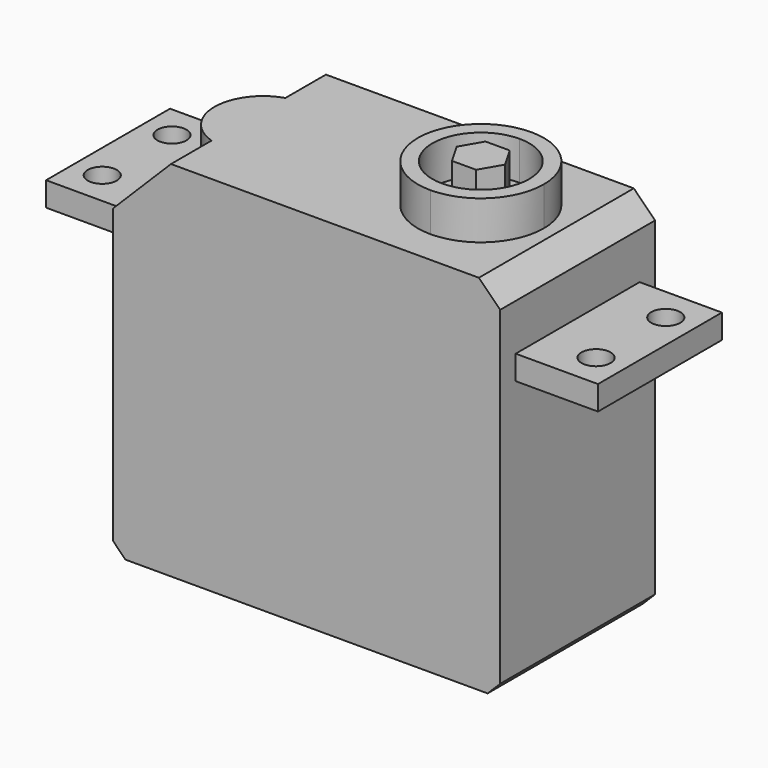
from build123d import *

# Parameters (mm, degrees)
F1_DEPTH    = 14
F2_DEPTH    = 13.5
F0_R        = 9.5
F3_DEPTH    = 9.5
F4_DEPTH    = 9.5
F5_DEPTH    = 28
F0_R_2      = 1.5
F6_DEPTH    = 2.5
F7_SIZE     = 2.2
F8_T1_DEPTH = 50.8601958556
F9_DEPTH    = 9.5
F10_SIZE    = 1.3


# Not quite as in the source:
# - a fillet or chamfer that OpenCascade refuses, or shapes differently, is made with other operations: its cross-section is extruded or revolved along the edge and cut away or added


with BuildPart() as f1:
    # F0 (on Top) → F1 (new body)
    with BuildSketch(Plane.XY):
        Polygon((10, 2.1650635095), (8.75, 2.1650635095), (7.5, 0), (8.75, -2.1650635095), (10, -2.1650635095), (10, 0), align=None)
        Polygon((11.25, 2.1650635095), (10, 2.1650635095), (10, 0), (10, -2.1650635095), (11.25, -2.1650635095), (12.5, 0), align=None)
    extrude(amount=F1_DEPTH)



with BuildPart() as f2:
    # F0 (on Top) → F2 (new body)
    with BuildSketch(Plane.XY):
        with BuildLine():
            ThreePointArc((10, -5), (5, 0), (10, 5))
            Line((10, 5), (10, 6.5))
            ThreePointArc((10, 6.5), (3.5, 0), (10, -6.5))
            Line((10, -6.5), (10, -5))
        make_face()
        with BuildLine():
            Line((10, 6.5), (10, 5))
            ThreePointArc((10, 5), (13.5355339059, 3.5355339059), (15, 0))
            ThreePointArc((15, 0), (13.5355339059, -3.5355339059), (10, -5))
            Line((10, -5), (10, -6.5))
            ThreePointArc((10, -6.5), (14.5961940777, -4.5961940777), (16.5, 0))
            ThreePointArc((16.5, 0), (14.5961940777, 4.5961940777), (10, 6.5))
        make_face()
    extrude(amount=F2_DEPTH)


with BuildPart() as f1_1:
    add(f1.part)

    add(f2.part)  # F3 merges F2
    # F0 (on Top) → F3 (join)
    with BuildSketch(Plane.XY):
        with Locations((10, 0)):
            Circle(F0_R)
        with BuildLine():
            ThreePointArc((10, -6.5), (3.5, 0), (10, 6.5))
            ThreePointArc((10, 6.5), (14.5961940777, 4.5961940777), (16.5, 0))
            ThreePointArc((16.5, 0), (14.5961940777, -4.5961940777), (10, -6.5))
        make_face(mode=Mode.SUBTRACT)
        with BuildLine():
            Line((7.5, 0), (8.75, 2.1650635095))
            Line((8.75, 2.1650635095), (10, 2.1650635095))
            Line((10, 2.1650635095), (10, 5))
            ThreePointArc((10, 5), (5, 0), (10, -5))
            Line((10, -5), (10, -2.1650635095))
            Line((10, -2.1650635095), (8.75, -2.1650635095))
            Line((8.75, -2.1650635095), (7.5, 0))
        make_face()
        with BuildLine():
            Line((10, 5), (10, 2.1650635095))
            Line((10, 2.1650635095), (11.25, 2.1650635095))
            Line((11.25, 2.1650635095), (12.5, 0))
            Line((12.5, 0), (11.25, -2.1650635095))
            Line((11.25, -2.1650635095), (10, -2.1650635095))
            Line((10, -2.1650635095), (10, -5))
            ThreePointArc((10, -5), (13.5355339059, -3.5355339059), (15, 0))
            ThreePointArc((15, 0), (13.5355339059, 3.5355339059), (10, 5))
        make_face()
    extrude(amount=F3_DEPTH)

    # F0 (on Top) → F4 (join)
    with BuildSketch(Plane.XY):
        Polygon((20, 10), (-20, 10), (-20, 8), (-20, 0), (-20, -8), (-20, -10), (20, -10), (20, -8), (20, 0), (20, 8), align=None)
        with BuildLine():
            ThreePointArc((-7.5, 0), (-12.5, -5), (-17.5, 0))
            ThreePointArc((-17.5, 0), (-12.5, 5), (-7.5, 0))
        make_face(mode=Mode.SUBTRACT)
        with Locations((10, 0)):
            Circle(F0_R, mode=Mode.SUBTRACT)
        with Locations((10, 0)):
            Circle(F0_R)
        with BuildLine():
            ThreePointArc((10, -6.5), (3.5, 0), (10, 6.5))
            ThreePointArc((10, 6.5), (14.5961940777, 4.5961940777), (16.5, 0))
            ThreePointArc((16.5, 0), (14.5961940777, -4.5961940777), (10, -6.5))
        make_face(mode=Mode.SUBTRACT)
    extrude(amount=F4_DEPTH)

    # F0 (on Top) → F5 (join)
    with BuildSketch(Plane.XY):
        Polygon((20, 10), (-20, 10), (-20, 8), (-20, 0), (-20, -8), (-20, -10), (20, -10), (20, -8), (20, 0), (20, 8), align=None)
        with BuildLine():
            ThreePointArc((-7.5, 0), (-12.5, -5), (-17.5, 0))
            ThreePointArc((-17.5, 0), (-12.5, 5), (-7.5, 0))
        make_face(mode=Mode.SUBTRACT)
        with Locations((10, 0)):
            Circle(F0_R, mode=Mode.SUBTRACT)
        with Locations((10, 0)):
            Circle(F0_R)
        with BuildLine():
            ThreePointArc((10, -6.5), (3.5, 0), (10, 6.5))
            ThreePointArc((10, 6.5), (14.5961940777, 4.5961940777), (16.5, 0))
            ThreePointArc((16.5, 0), (14.5961940777, -4.5961940777), (10, -6.5))
        make_face(mode=Mode.SUBTRACT)
        Polygon((10, 2.1650635095), (8.75, 2.1650635095), (7.5, 0), (8.75, -2.1650635095), (10, -2.1650635095), (10, 0), align=None)
        Polygon((11.25, 2.1650635095), (10, 2.1650635095), (10, 0), (10, -2.1650635095), (11.25, -2.1650635095), (12.5, 0), align=None)
        with BuildLine():
            Line((7.5, 0), (8.75, 2.1650635095))
            Line((8.75, 2.1650635095), (10, 2.1650635095))
            Line((10, 2.1650635095), (10, 5))
            ThreePointArc((10, 5), (5, 0), (10, -5))
            Line((10, -5), (10, -2.1650635095))
            Line((10, -2.1650635095), (8.75, -2.1650635095))
            Line((8.75, -2.1650635095), (7.5, 0))
        make_face()
        with BuildLine():
            Line((10, 5), (10, 2.1650635095))
            Line((10, 2.1650635095), (11.25, 2.1650635095))
            Line((11.25, 2.1650635095), (12.5, 0))
            Line((12.5, 0), (11.25, -2.1650635095))
            Line((11.25, -2.1650635095), (10, -2.1650635095))
            Line((10, -2.1650635095), (10, -5))
            ThreePointArc((10, -5), (13.5355339059, -3.5355339059), (15, 0))
            ThreePointArc((15, 0), (13.5355339059, 3.5355339059), (10, 5))
        make_face()
        with BuildLine():
            ThreePointArc((10, -5), (5, 0), (10, 5))
            Line((10, 5), (10, 6.5))
            ThreePointArc((10, 6.5), (3.5, 0), (10, -6.5))
            Line((10, -6.5), (10, -5))
        make_face()
        with BuildLine():
            Line((10, 6.5), (10, 5))
            ThreePointArc((10, 5), (13.5355339059, 3.5355339059), (15, 0))
            ThreePointArc((15, 0), (13.5355339059, -3.5355339059), (10, -5))
            Line((10, -5), (10, -6.5))
            ThreePointArc((10, -6.5), (14.5961940777, -4.5961940777), (16.5, 0))
            ThreePointArc((16.5, 0), (14.5961940777, 4.5961940777), (10, 6.5))
        make_face()
        with BuildLine():
            ThreePointArc((-7.5, 0), (-12.5, 5), (-17.5, 0))
            ThreePointArc((-17.5, 0), (-12.5, -5), (-7.5, 0))
        make_face()
    extrude(amount=-F5_DEPTH)

    # F0 (on Top) → F6 (join)
    with BuildSketch(Plane.XY):
        Polygon((28.5, 8), (20, 8), (20, 0), (20, -8), (28.5, -8), align=None)
        with Locations((25.5, -4.5)):
            Circle(F0_R_2, mode=Mode.SUBTRACT)
        with Locations((25.5, 4.5)):
            Circle(F0_R_2, mode=Mode.SUBTRACT)
        Polygon((-20, 0), (-20, 8), (-28.5, 8), (-28.5, -8), (-20, -8), align=None)
        with Locations((-25.5, -4.5)):
            Circle(F0_R_2, mode=Mode.SUBTRACT)
        with Locations((-25.5, 4.5)):
            Circle(F0_R_2, mode=Mode.SUBTRACT)
    extrude(amount=F6_DEPTH)

    # F7
    f7_edges = [f1_1.edges().sort_by_distance(p)[0] for p in [
        (20, 0, 9.5),
    ]]
    chamfer(f7_edges, length=F7_SIZE)

    # F8: chamfer of 6 on 1 edges, made by hand

    # F8_s2 → F8_t1 (cut)
    with BuildSketch(Plane.XZ.offset(-25.4300979278)):
        Polygon((-14, 9.5), (-20, 3.5), (-20, 9.5), align=None)
    extrude(amount=F8_T1_DEPTH, mode=Mode.SUBTRACT)

    # F0 (on Top) → F9 (join)
    with BuildSketch(Plane.XY):
        with BuildLine():
            ThreePointArc((-7.5, 0), (-12.5, 5), (-17.5, 0))
            ThreePointArc((-17.5, 0), (-12.5, -5), (-7.5, 0))
        make_face()
    extrude(amount=F9_DEPTH)

    # F10
    f10_edges = [f1_1.edges().sort_by_distance(p)[0] for p in [
        (20, 0, -28),
        (-20, 0, -28),
    ]]
    chamfer(f10_edges, length=F10_SIZE)


solid = f1_1.part
